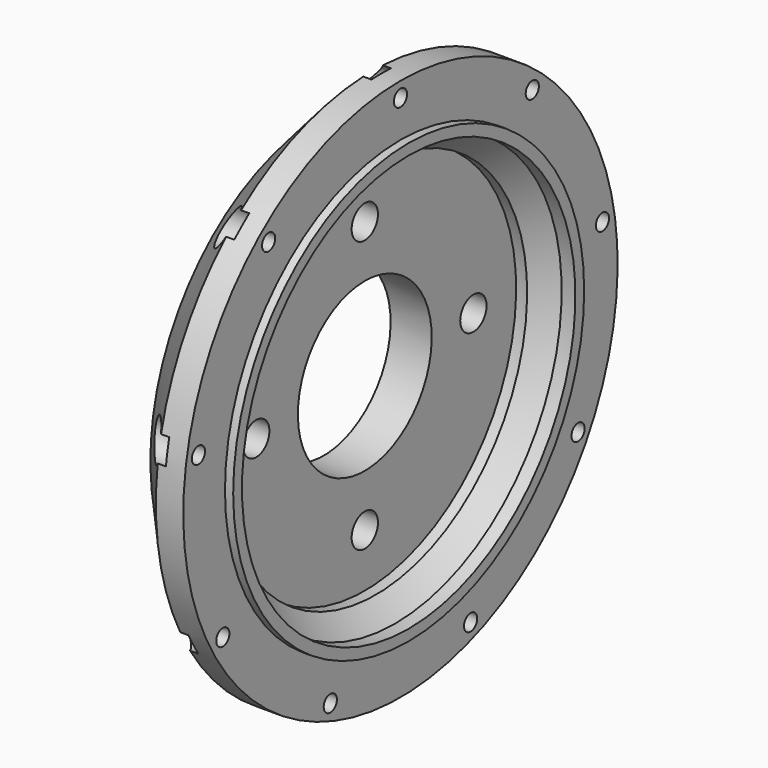
from build123d import *

# Parameters (mm, degrees)
F3_R             = 6
F4_DEPTH         = 31
F4_COPIES_COUNT  = 4
F6_R             = 3
F7_DEPTH         = 31
F7_COPIES_COUNT  = 9
F9_R             = 7
F10_DEPTH        = 21
F10_COPIES_COUNT = 9


# Not quite as in the source:
# - a pattern or mirror of a feature is missing from the dataset's text; its kind, count and spacing are read off the source's solid


with BuildPart() as f1:
    # F0 (on Front) → F1 (revolve)
    with BuildSketch(Plane.XZ):
        Polygon((-5, 76), (0, 76), (0, 80), (-3, 80), (-5, 80), align=None)
        Polygon((-12, 69), (-5, 76), (-5, 80), (-3, 80), (-3, 99), (-13, 99), (-31, 79), (-31, 30.5), (-16, 30.5), (-16, 69), align=None)
    revolve(axis=Axis((-15.5, 0, 0), (-1, 0, 0)))

    # F3 (on offset) → F4 (cut)
    with BuildSketch(Plane.YZ.offset(-16)):
        with Locations((0, 49.5)):
            Circle(F3_R)
    f4 = extrude(amount=-F4_DEPTH, mode=Mode.SUBTRACT)

    # F4_copies: F4 ×4 about axis
    f4_copies_axis = Axis((0, 0, 0), (1, 0, 0))
    for i in range(1, F4_COPIES_COUNT):
        add(f4.rotate(f4_copies_axis, i * 360 / F4_COPIES_COUNT), mode=Mode.SUBTRACT)

    # F6 (on offset) → F7 (cut)
    with BuildSketch(Plane.YZ.offset(-3)):
        with Locations((0, 93.5)):
            Circle(F6_R)
    f7 = extrude(amount=-F7_DEPTH, mode=Mode.SUBTRACT)

    # F7_copies: F7 ×9 about axis
    f7_copies_axis = Axis((0, 0, 0), (1, 0, 0))
    for i in range(1, F7_COPIES_COUNT):
        add(f7.rotate(f7_copies_axis, i * 360 / F7_COPIES_COUNT), mode=Mode.SUBTRACT)

    # F9 (on offset) → F10 (cut)
    with BuildSketch(Plane.YZ.offset(-10)):
        with Locations((0, 93.5)):
            Circle(F9_R)
    f10 = extrude(amount=-F10_DEPTH, mode=Mode.SUBTRACT)

    # F10_copies: F10 ×9 about axis
    f10_copies_axis = Axis((0, 0, 0), (1, 0, 0))
    for i in range(1, F10_COPIES_COUNT):
        add(f10.rotate(f10_copies_axis, i * 360 / F10_COPIES_COUNT), mode=Mode.SUBTRACT)


solid = f1.part
